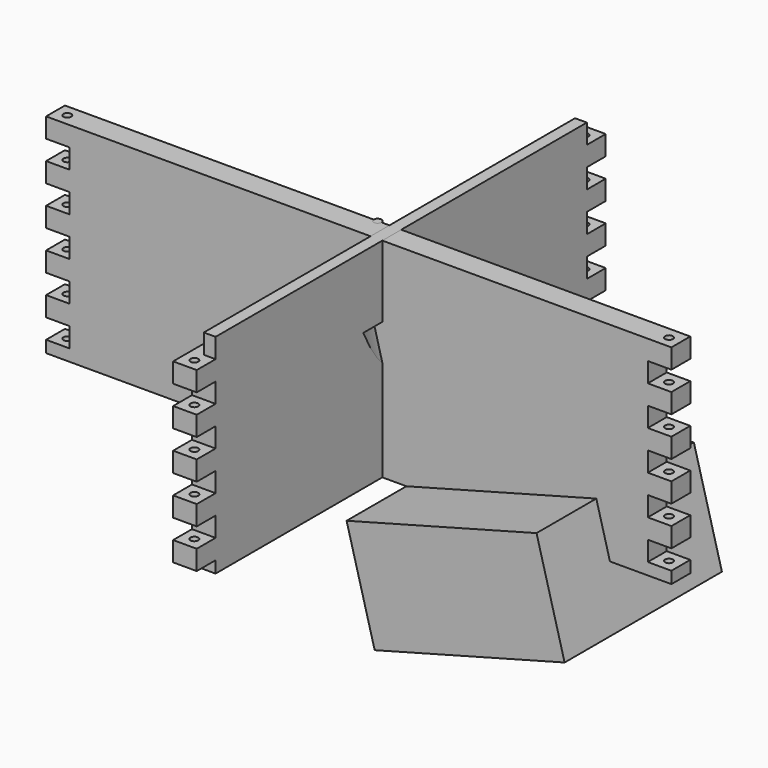
from build123d import *

# Parameters (mm, degrees)
F1_DEPTH  = 19.05
F3_DEPTH  = 19.05
F4_W      = 9.525
F4_H      = 15.875
F5_DEPTH  = 381
F6_R      = 3.175
F7_DEPTH  = 152.4
F8_R      = 3.175
F9_DEPTH  = 177.8
F10_R     = 3.175
F11_DEPTH = 168.275
F13_DEPTH = 79.375
F15_DEPTH = 111.76


with BuildPart() as f1:
    # F0 (on Front) → F1 (new body)
    with BuildSketch(Plane.XZ):
        Polygon((252.4125, 168.275), (0, 168.275), (-252.4125, 168.275), (-252.4125, 152.4), (-233.3625, 152.4), (-233.3625, 136.525), (-252.4125, 136.525), (-252.4125, 120.65), (-233.3625, 120.65), (-233.3625, 104.775), (-252.4125, 104.775), (-252.4125, 88.9), (-233.3625, 88.9), (-233.3625, 73.025), (-252.4125, 73.025), (-252.4125, 57.15), (-233.3625, 57.15), (-233.3625, 41.275), (-252.4125, 41.275), (-252.4125, 25.4), (-233.3625, 25.4), (-233.3625, 9.525), (-252.4125, 9.525), (-252.4125, 0), (0, 0), (252.4125, 0), (252.4125, 9.525), (233.3625, 9.525), (233.3625, 25.4), (252.4125, 25.4), (252.4125, 41.275), (233.3625, 41.275), (233.3625, 57.15), (252.4125, 57.15), (252.4125, 73.025), (233.3625, 73.025), (233.3625, 88.9), (252.4125, 88.9), (252.4125, 104.775), (233.3625, 104.775), (233.3625, 120.65), (252.4125, 120.65), (252.4125, 136.525), (233.3625, 136.525), (233.3625, 152.4), (252.4125, 152.4), align=None)
    extrude(amount=F1_DEPTH)

    # F8 (on face) → F9 (cut)
    with BuildSketch(Plane.XY.offset(168.275)):
        with Locations((-242.8875, -9.525)):
            Circle(F8_R)
        with Locations((242.8875, -9.525)):
            Circle(F8_R)
    extrude(amount=-F9_DEPTH, mode=Mode.SUBTRACT)


with BuildPart() as f3:
    # F2 (on Right) → F3 (new body)
    with BuildSketch(Plane.YZ):
        Polygon((187.325, 168.275), (0, 168.275), (-187.325, 168.275), (-187.325, 152.4), (-206.375, 152.4), (-206.375, 136.525), (-187.325, 136.525), (-187.325, 120.65), (-206.375, 120.65), (-206.375, 104.775), (-187.325, 104.775), (-187.325, 88.9), (-206.375, 88.9), (-206.375, 73.025), (-187.325, 73.025), (-187.325, 57.15), (-206.375, 57.15), (-206.375, 41.275), (-187.325, 41.275), (-187.325, 25.4), (-206.375, 25.4), (-206.375, 9.525), (-187.325, 9.525), (-187.325, 0), (0, 0), (187.325, 0), (187.325, 9.525), (206.375, 9.525), (206.375, 25.4), (187.325, 25.4), (187.325, 41.275), (206.375, 41.275), (206.375, 57.15), (187.325, 57.15), (187.325, 73.025), (206.375, 73.025), (206.375, 88.9), (187.325, 88.9), (187.325, 104.775), (206.375, 104.775), (206.375, 120.65), (187.325, 120.65), (187.325, 136.525), (206.375, 136.525), (206.375, 152.4), (187.325, 152.4), align=None)
    extrude(amount=F3_DEPTH)

    # F4 (on face) → F5 (cut)
    with BuildSketch(Plane.XZ.offset(187.325)):
        with Locations((4.7625, 160.3375)):
            Rectangle(F4_W, F4_H)
    extrude(amount=-F5_DEPTH, mode=Mode.SUBTRACT)

    # F6 (on face) → F7 (cut)
    with BuildSketch(Plane.XY.offset(152.4)):
        with Locations((9.525, 196.85)):
            Circle(F6_R)
        with Locations((9.525, -196.85)):
            Circle(F6_R)
    extrude(amount=-F7_DEPTH, mode=Mode.SUBTRACT)

    # F14 (on face) → F15 (cut)
    with BuildSketch(Plane(origin=(2.5756693374, 0, -9.6125288307), x_dir=(0.9659258263, 0, 0.2588190451), z_dir=(-0.2588190451, 0, 0.9659258263))):
        with BuildLine():
            ThreePointArc((116.5149594142, -79.375), (172.6415601709, -56.1266007567), (195.8899594142, 0))
            ThreePointArc((195.8899594142, 0), (172.6415601709, 56.1266007567), (116.5149594142, 79.375))
            ThreePointArc((116.5149594142, 79.375), (60.3883587272, 56.1266008263), (37.1399594142, 1.97e-07))
            ThreePointArc((37.1399594142, 1.97e-07), (60.3883585879, -56.126600687), (116.5149594142, -79.375))
        make_face()
    extrude(amount=F15_DEPTH, mode=Mode.SUBTRACT)


with BuildPart() as f11:
    # F10 (on Top) → F11 (new body)
    with BuildSketch(Plane.XY):
        Circle(F10_R)
    extrude(amount=F11_DEPTH)


with BuildPart() as f13:
    # F12 (on Front) → F13 (new body, symmetric)
    with BuildSketch(Plane.XZ):
        Polygon((191.7908402463, 41.08752341), (38.4501153229, 0), (61.120134133, -84.6056620075), (214.4608590563, -43.5181385975), align=None)
    extrude(amount=F13_DEPTH, both=True)


solid = Compound([f1.part, f3.part, f11.part, f13.part])
